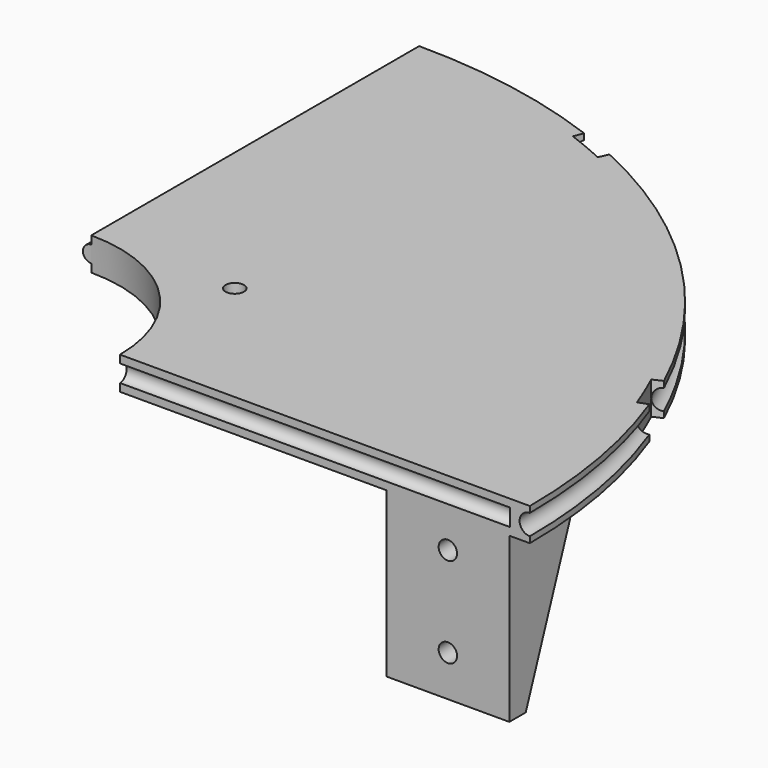
from build123d import *

# Parameters (mm, degrees)
F0_R      = 2.25
F1_DEPTH  = 8
F4_R      = 2.5
F6_W      = 30
F6_H      = 20
F6_W_2    = 20
F6_H_2    = 30
F7_DEPTH  = 40
F8_W      = 18
F8_H      = 15
F8_W_2    = 15
F8_H_2    = 18
F9_DEPTH  = 40
F10_SIZE2 = 39.99999
F10_SIZE  = 14.99999
F11_R     = 2.25
F12_DEPTH = 25
F13_SIZE2 = 14.99999
F13_SIZE  = 39.99999
F14_R     = 2.25
F15_DEPTH = 25
F17_DEPTH = 25
F20_R     = 2
F23_DEPTH = 48.001
F24_R     = 2.1
F27_DEPTH = 6
F29_DEPTH = 6
F30_SIZE2 = 14.99999
F30_SIZE  = 45.99999
F31_SIZE2 = 14.99999
F31_SIZE  = 45.99999
F32_R     = 2


# Not quite as in the source:
# - a fillet or chamfer is up to 0.001 mm smaller than in the source, because OpenCascade refuses the exact size


with BuildPart() as f1:
    # F0 (on Top) → F1 (new body)
    with BuildSketch(Plane.XY):
        with BuildLine():
            Line((35, 0), (135, 0))
            ThreePointArc((135, 0), (95.4594154602, 95.4594154602), (0, 135))
            Line((0, 135), (0, 35))
            ThreePointArc((0, 35), (24.7487373415, 24.7487373415), (35, 0))
        make_face()
        with Locations((35, 35)):
            Circle(F0_R, mode=Mode.SUBTRACT)
    extrude(amount=F1_DEPTH)

    # F5: sweep along a path in F3
    with BuildLine(Plane.XY.offset(4)) as f5_path:
        CenterArc((0, 0), 135, 0, 360)
    # F4 (on face) → F5 (sweep, cut)
    with BuildSketch(Plane.XZ):
        with Locations((135, 4)):
            Circle(F4_R)
    sweep(path=f5_path.line, mode=Mode.SUBTRACT)

    # F6 (on face) → F7 (join)
    with BuildSketch(Plane(origin=(0, 0, 0), x_dir=(1, 0, 0), z_dir=(0, 0, -1))):
        with Locations((115, -10)):
            Rectangle(F6_W, F6_H)
        with Locations((10, -115)):
            Rectangle(F6_W_2, F6_H_2)
    extrude(amount=F7_DEPTH)

    # F8 (on face) → F9 (cut)
    with BuildSketch(Plane(origin=(0, 0, -40), x_dir=(1, 0, 0), z_dir=(0, 0, -1))):
        with Locations((115, -12.5)):
            Rectangle(F8_W, F8_H)
        with Locations((12.5, -115)):
            Rectangle(F8_W_2, F8_H_2)
    extrude(amount=-F9_DEPTH, mode=Mode.SUBTRACT)

    # F10 (size 15 and 40 in the source; OpenCascade refuses exactly that, so slightly less here)
    f10_edges = [f1.edges().sort_by_distance(p)[0] for p in [
        (127, 20, -40),
    ]]
    f10_side = f1.faces().sort_by_distance((129.639445, 10, -40))[0]
    chamfer(f10_edges, length=F10_SIZE, length2=F10_SIZE2, reference=f10_side)

    # F11 (on face) → F12 (cut)
    with BuildSketch(Plane(origin=(0, 5, 0), x_dir=(-1, 0, 0), z_dir=(0, 1, 0))):
        with Locations((-115, -8)):
            Circle(F11_R)
        with Locations((-115, -30)):
            Circle(F11_R)
    extrude(amount=-F12_DEPTH, mode=Mode.SUBTRACT)

    # F13 (size 40 and 15 in the source; OpenCascade refuses exactly that, so slightly less here)
    f13_edges = [f1.edges().sort_by_distance(p)[0] for p in [
        (20, 127, -40),
    ]]
    chamfer(f13_edges, length=F13_SIZE, length2=F13_SIZE2)

    # F14 (on face) → F15 (cut)
    with BuildSketch(Plane.YZ.offset(5)):
        with Locations((115, -30)):
            Circle(F14_R)
        with Locations((113.5, -8)):
            Circle(F14_R)
    extrude(amount=-F15_DEPTH, mode=Mode.SUBTRACT)

    # F16 (on face) → F17 (cut)
    with BuildSketch(Plane.XY.offset(8)):
        with BuildLine():
            ThreePointArc((120.4496071259, 55.2099822787), (122.4117800348, 50.7110057948), (124.2059779255, 46.1424430169))
            Line((124.2059779255, 46.1424430169), (126.549486943, 47.0130551493))
            ThreePointArc((126.549486943, 47.0130551493), (124.7214362618, 51.6678172249), (122.7222412226, 56.2516800575))
            Line((122.7222412226, 56.2516800575), (120.4496071259, 55.2099822787))
        make_face()
        with BuildLine():
            Line((47.0017845491, 126.5536733928), (46.1313811315, 124.2100868484))
            ThreePointArc((46.1313811315, 124.2100868484), (50.7001036814, 122.416295838), (55.1992548973, 120.4545236128))
            Line((55.1992548973, 120.4545236128), (56.2407502727, 122.7272504734))
            ThreePointArc((56.2407502727, 122.7272504734), (51.6567094112, 124.7260372689), (47.0017845491, 126.5536733928))
        make_face()
    extrude(amount=-F17_DEPTH, mode=Mode.SUBTRACT)

    # F21: sweep along a path in F19
    with BuildLine(Plane(origin=(0, 0, 0), x_dir=(0, -1, 0), z_dir=(-1, 0, 0))) as f21_path:
        Line((-130, 4), (0, 4))
    # F20 (on Front) → F21 (sweep)
    with BuildSketch(Plane.XZ):
        with Locations((0, 4)):
            Circle(F20_R)
    sweep(path=f21_path.line)

    # F22 (on face) → F23 (cut, through all)
    with BuildSketch(Plane.XY.offset(8)):
        with BuildLine():
            ThreePointArc((0, 35), (-24.7487373415, -24.7487373415), (35, 0))
            ThreePointArc((35, 0), (24.7487373415, 24.7487373415), (0, 35))
        make_face()
    extrude(amount=-F23_DEPTH, mode=Mode.SUBTRACT)

    # F25: sweep along a path in F18
    with BuildLine(Plane.XZ) as f25_path:
        Line((0, 4), (130.2, 4))
    # F24 (on Right) → F25 (sweep, cut)
    with BuildSketch(Plane.YZ):
        with Locations((0, 4)):
            Circle(F24_R)
    sweep(path=f25_path.line, mode=Mode.SUBTRACT)

    # F26 (on face) → F27 (cut)
    with BuildSketch(Plane(origin=(0, 0, 0), x_dir=(1, 0, 0), z_dir=(0, 0, -1))):
        with BuildLine():
            Line((37, -40), (7, -40))
            ThreePointArc((7, -40), (5.5857864376, -40.5857864376), (5, -42))
            Line((5, -42), (5, -100))
            Line((5, -100), (20, -100))
            Line((20, -100), (20, -106))
            Line((20, -106), (5, -106))
            Line((5, -106), (5, -124))
            Line((5, -124), (20, -124))
            ThreePointArc((20, -124), (88.8144132447, -88.8144132447), (124, -20))
            Line((124, -20), (124, -5))
            Line((124, -5), (106, -5))
            Line((106, -5), (106, -20))
            Line((106, -20), (100, -20))
            Line((100, -20), (100, -5))
            Line((100, -5), (42, -5))
            ThreePointArc((42, -5), (40.5857864376, -5.5857864376), (40, -7))
            Line((40, -7), (40, -37))
            ThreePointArc((40, -37), (39.1213203436, -39.1213203436), (37, -40))
        make_face()
    extrude(amount=-F27_DEPTH, mode=Mode.SUBTRACT)

    # F28 (on face) → F29 (cut)
    with BuildSketch(Plane(origin=(0, 0, 0), x_dir=(1, 0, 0), z_dir=(0, 0, -1))):
        with BuildLine():
            ThreePointArc((35.5519480519, -11.9293331629), (26.5165042945, -26.5165042945), (11.9293331629, -35.5519480519))
            ThreePointArc((11.9293331629, -35.5519480519), (11.2605211715, -36.6611645928), (12.2474487139, -37.5))
            Line((12.2474487139, -37.5), (29.4490991722, -37.5))
            ThreePointArc((29.4490991722, -37.5), (30.2430984056, -37.1079187589), (30.4144732292, -36.2391304348))
            ThreePointArc((30.4144732292, -36.2391304348), (31.6412427894, -31.6412427894), (36.2391304348, -30.4144732292))
            ThreePointArc((36.2391304348, -30.4144732292), (37.1079187589, -30.2430984056), (37.5, -29.4490991722))
            Line((37.5, -29.4490991722), (37.5, -12.2474487139))
            ThreePointArc((37.5, -12.2474487139), (36.6611645928, -11.2605211715), (35.5519480519, -11.9293331629))
        make_face()
    extrude(amount=-F29_DEPTH, mode=Mode.SUBTRACT)

    # F30 (size 46 and 15 in the source; OpenCascade refuses exactly that, so slightly less here)
    f30_edges = [f1.edges().sort_by_distance(p)[0] for p in [
        (20, 103, -40),
    ]]
    f30_side = f1.faces().sort_by_distance((20, 103, -17))[0]
    chamfer(f30_edges, length=F30_SIZE, length2=F30_SIZE2, reference=f30_side)

    # F31 (size 46 and 15 in the source; OpenCascade refuses exactly that, so slightly less here)
    f31_edges = [f1.edges().sort_by_distance(p)[0] for p in [
        (103, 20, -40),
    ]]
    f31_side = f1.faces().sort_by_distance((103, 20, -17))[0]
    chamfer(f31_edges, length=F31_SIZE, length2=F31_SIZE2, reference=f31_side)

    # F32
    f32_edges = [f1.edges().sort_by_distance(p)[0] for p in [
        (5, 100, 3),
        (100, 5, 3),
    ]]
    fillet(f32_edges, radius=F32_R)


solid = f1.part
